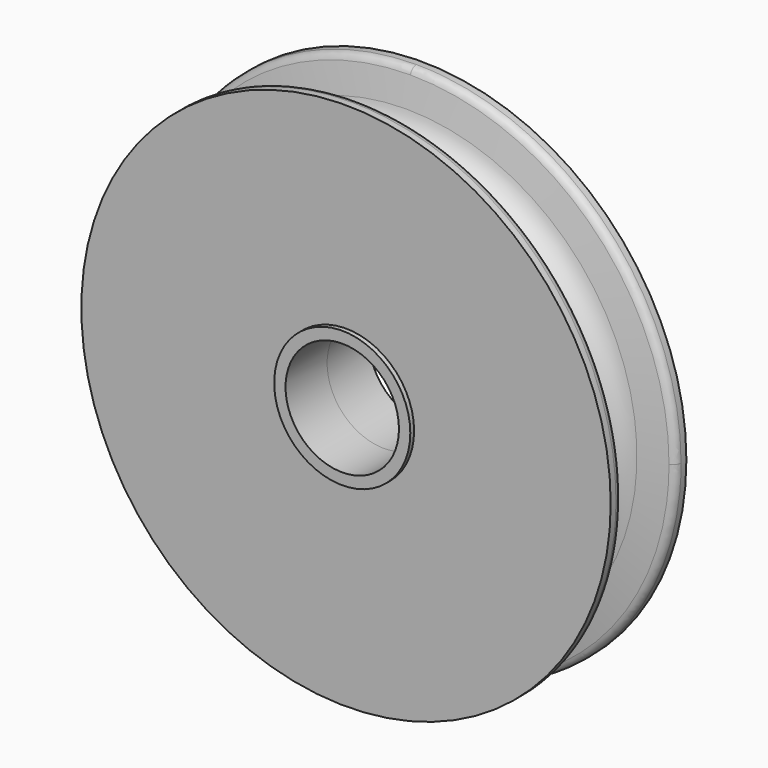
from build123d import *

# Parameters (mm, degrees)
F0_R          = 11.43
F0_R_2        = 9.525
F1_DEPTH      = 8.73125
F1_DEPTH_BACK = 8.7376
F0_R_3        = 44.45
F2_DEPTH      = 7.9375
F2_DEPTH_BACK = 7.9502
F5_R          = 1.27


with BuildPart() as f1:
    # F0 (on Front) → F1 (new body, two sides)
    with BuildSketch(Plane.XZ) as f1_sk:
        Circle(F0_R)
        Circle(F0_R_2, mode=Mode.SUBTRACT)
    extrude(amount=F1_DEPTH)
    extrude(f1_sk.sketch, amount=-F1_DEPTH_BACK)

    # F0 (on Front) → F2 (join, two sides)
    with BuildSketch(Plane.XZ) as f2_sk:
        Circle(F0_R_3)
        Circle(F0_R, mode=Mode.SUBTRACT)
    extrude(amount=F2_DEPTH)
    extrude(f2_sk.sketch, amount=-F2_DEPTH_BACK)

    # F3 (on Right) → F4 (revolve, cut)
    with BuildSketch(Plane.YZ):
        with BuildLine():
            Line((-6.35, 47.3075), (-4.6732280163, 38.7697058197))
            ThreePointArc((-4.6732280163, 38.7697058197), (0, 34.925), (4.6732280163, 38.7697058197))
            Line((4.6732280163, 38.7697058197), (6.35, 47.3075))
            Line((6.35, 47.3075), (0, 47.3075))
            Line((0, 47.3075), (-6.35, 47.3075))
        make_face()
    revolve(axis=Axis((0, 33.8884852827, 0), (0, 1, 0)), mode=Mode.SUBTRACT)

    # F5
    f5_edges = [f1.edges().sort_by_distance(p)[0] for p in [
        (31.430896, 5.788804, 31.430896),
        (-31.430896, 5.788804, -31.430896),
        (-31.430896, -5.788804, -31.430896),
        (31.430896, -5.788804, 31.430896),
    ]]
    fillet(f5_edges, radius=F5_R)


solid = f1.part
